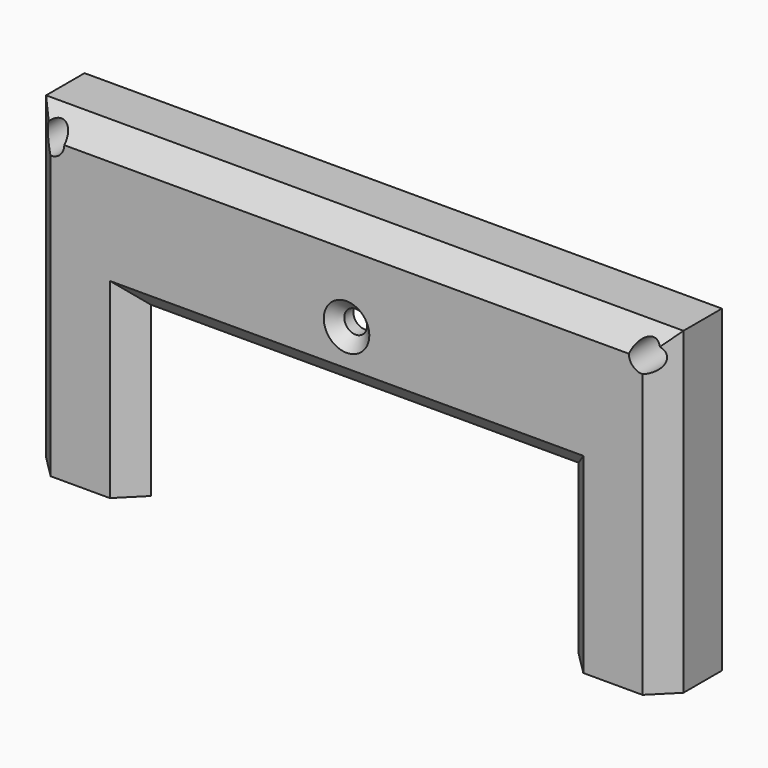
from build123d import *

# Parameters (mm, degrees)
F0_W        = 140
F0_H        = 252.5
F0_R        = 1
F0_W_2      = 94
F0_H_2      = 152.5
F0_R_2      = 2.5
F0_W_3      = 12
F0_H_3      = 34
F1_DEPTH    = 15.56
F2_DEPTH    = 10.56
F3_T1_DEPTH = 165.7168298797
F3_T3_DEPTH = 278.2168298797
F4_SIZE     = 2.5
F5_R        = 3
F6_DEPTH    = 10
F7_SIZE     = 4.99999
F8_W        = 161.2529857084
F8_H        = 182.5
F9_DEPTH    = 25
F11_W       = 6
F11_H       = 50
F12_DEPTH   = 6


# Not quite as in the source:
# - a fillet or chamfer that OpenCascade refuses, or shapes differently, is made with other operations: its cross-section is extruded or revolved along the edge and cut away or added
# - a fillet or chamfer is up to 0.001 mm smaller than in the source, because OpenCascade refuses the exact size
# - a feature names something its author has since deleted; it is built from what else it names


with BuildPart() as f1:
    # F0 (on Front) → F1 (new body)
    with BuildSketch(Plane.XZ):
        with Locations((-70, 126.25)):
            Rectangle(F0_W, F0_H)
        with Locations((-135, 5)):
            Circle(F0_R, mode=Mode.SUBTRACT)
        with Locations((-5, 5)):
            Circle(F0_R, mode=Mode.SUBTRACT)
        with Locations((-135, 247.5)):
            Circle(F0_R, mode=Mode.SUBTRACT)
        Polygon((-130, 44), (-130, 242.5), (-10, 242.5), (-10, 44), (-64, 44), (-64, 10), (-76, 10), (-76, 44), align=None, mode=Mode.SUBTRACT)
        with Locations((-5, 247.5)):
            Circle(F0_R, mode=Mode.SUBTRACT)
        Polygon((-10, 242.5), (-130, 242.5), (-130, 44), (-76, 44), (-64, 44), (-10, 44), align=None)
        with Locations((-70, 143.25)):
            Rectangle(F0_W_2, F0_H_2, mode=Mode.SUBTRACT)
        with Locations((-70, 232.5)):
            Circle(F0_R_2, mode=Mode.SUBTRACT)
        with Locations((-70, 27)):
            Rectangle(F0_W_3, F0_H_3)
    extrude(amount=F1_DEPTH)

    # F0 (on Front) → F2 (cut)
    with BuildSketch(Plane.XZ):
        Polygon((-10, 242.5), (-130, 242.5), (-130, 44), (-76, 44), (-64, 44), (-10, 44), align=None)
        with Locations((-70, 143.25)):
            Rectangle(F0_W_2, F0_H_2, mode=Mode.SUBTRACT)
        with Locations((-70, 232.5)):
            Circle(F0_R_2, mode=Mode.SUBTRACT)
        with Locations((-70, 27)):
            Rectangle(F0_W_3, F0_H_3)
    extrude(amount=F2_DEPTH, mode=Mode.SUBTRACT)

    # F3: chamfer of 5 on 4 edges, made by hand

    # F3_s2 → F3_t1 (cut)
    with BuildSketch(Plane.YZ.offset(-152.8584149398)):
        Polygon((-10.56, 0), (-15.56, 5), (-15.56, 0), align=None)
        Polygon((-15.56, 247.5), (-10.56, 252.5), (-15.56, 252.5), align=None)
    extrude(amount=F3_T1_DEPTH, mode=Mode.SUBTRACT)

    # F3_s4 → F3_t3 (cut)
    with BuildSketch(Plane.XY.offset(-12.8584149398)):
        Polygon((-140, -10.56), (-135, -15.56), (-140, -15.56), align=None)
        Polygon((0, -10.56), (-5, -15.56), (0, -15.56), align=None)
    extrude(amount=F3_T3_DEPTH, mode=Mode.SUBTRACT)

    # F4
    f4_edges = [f1.edges().sort_by_distance(p)[0] for p in [
        (-72.5, -15.56, 232.5),
    ]]
    chamfer(f4_edges, length=F4_SIZE)

    # F5 (on face) → F6 (cut)
    with BuildSketch(Plane.XZ.offset(15.56)):
        with Locations((-135, 247.5)):
            Circle(F5_R)
        with Locations((-135, 5)):
            Circle(F5_R)
        with Locations((-5, 247.5)):
            Circle(F5_R)
        with Locations((-5, 5)):
            Circle(F5_R)
    extrude(amount=-F6_DEPTH, mode=Mode.SUBTRACT)

    # F7 (size 5 in the source; OpenCascade refuses exactly that, so slightly less here)
    f7_edges = [f1.edges().sort_by_distance(p)[0] for p in [
        (-70, -15.56, 67),
        (-117, -15.56, 143.25),
        (-23, -15.56, 143.25),
        (-70, -15.56, 219.5),
    ]]
    chamfer(f7_edges, length=F7_SIZE)

    # F8 (on face) → F9 (cut)
    with BuildSketch(Plane.XZ.offset(15.56)):
        with Locations((-74.815297965, 91.25)):
            Rectangle(F8_W, F8_H)
    extrude(amount=-F9_DEPTH, mode=Mode.SUBTRACT)

    # F11 (on offset) → F12 (cut)
    with BuildSketch(Plane(origin=(0, -2.5, 0), x_dir=(-1, 0, 0), z_dir=(0, 1, 0))):
        with Locations((135, 182.5)):
            Rectangle(F11_W, F11_H)
        with Locations((5, 182.5)):
            Rectangle(F11_W, F11_H)
    extrude(amount=-F12_DEPTH, mode=Mode.SUBTRACT)


solid = f1.part
